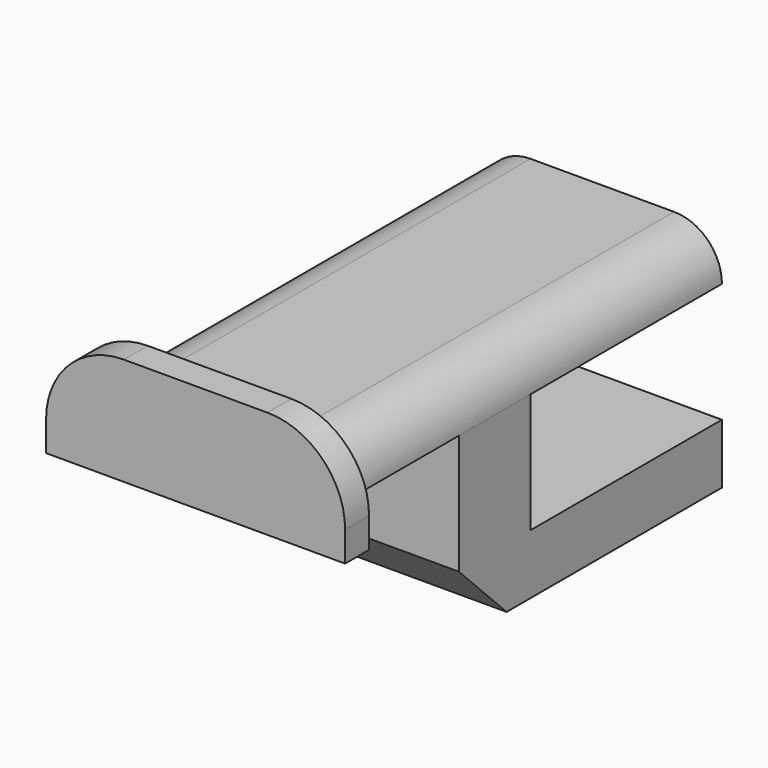
from build123d import *

# Parameters (mm, degrees)
F0_W      = 40
F0_H      = 80
F1_DEPTH  = 8
F2_W      = 40
F2_H      = 15
F3_DEPTH  = 30
F4_W      = 40
F4_H      = 10
F5_DEPTH  = 40
F6_R      = 7.99999
F7_SIZE2  = 10
F7_SIZE   = 10
F9_DEPTH  = 5
F10_W     = 48
F10_H     = 5
F10_W_2   = 1
F11_DEPTH = 5


# Not quite as in the source:
# - a fillet or chamfer is up to 0.001 mm smaller than in the source, because OpenCascade refuses the exact size


with BuildPart() as f1:
    # F0 (on Top) → F1 (new body)
    with BuildSketch(Plane.XY):
        with Locations((-20, 2.0996452868)):
            Rectangle(F0_W, F0_H)
    extrude(amount=F1_DEPTH)

    # F2 (on face) → F3 (join)
    with BuildSketch(Plane(origin=(0, 0, 0), x_dir=(1, 0, 0), z_dir=(0, 0, -1))):
        with Locations((-20, 5.4003547132)):
            Rectangle(F2_W, F2_H)
    extrude(amount=F3_DEPTH)

    # F4 (on face) → F5 (join)
    with BuildSketch(Plane(origin=(0, 2.0996452868, 0), x_dir=(-1, 0, 0), z_dir=(0, 1, 0))):
        with Locations((20, -25)):
            Rectangle(F4_W, F4_H)
    extrude(amount=F5_DEPTH)

    # F6 (radius 8 in the source; OpenCascade refuses exactly that, so slightly less here)
    f6_edges = [f1.edges().sort_by_distance(p)[0] for p in [
        (0, 2.099645, 8),
        (-40, 2.099645, 8),
    ]]
    fillet(f6_edges, radius=F6_R)

    # F7
    f7_edges = [f1.edges().sort_by_distance(p)[0] for p in [
        (-20, -12.900355, -30),
    ]]
    chamfer(f7_edges, length=F7_SIZE, length2=F7_SIZE2)

    # F8 (on face) → F9 (join)
    with BuildSketch(Plane.XZ.offset(37.9003547132)):
        with BuildLine():
            Line((-44, -5), (4, -5))
            ThreePointArc((4, -5), (2.8166538264, 7.2111025509), (-8, 13))
            Line((-8, 13), (-32, 13))
            ThreePointArc((-32, 13), (-42.8166538264, 7.2111025509), (-44, -5))
        make_face()
    extrude(amount=F9_DEPTH)

    # F10 (on face) → F11 (join)
    with BuildSketch(Plane(origin=(0, 0, -5), x_dir=(1, 0, 0), z_dir=(0, 0, -1))):
        with Locations((-20, 40.4003547132)):
            Rectangle(F10_W, F10_H)
        with Locations((-44.5, 40.4003547132)):
            Rectangle(F10_W_2, F10_H)
        with Locations((4.5, 40.4003547132)):
            Rectangle(F10_W_2, F10_H)
    extrude(amount=-F11_DEPTH)


solid = f1.part
